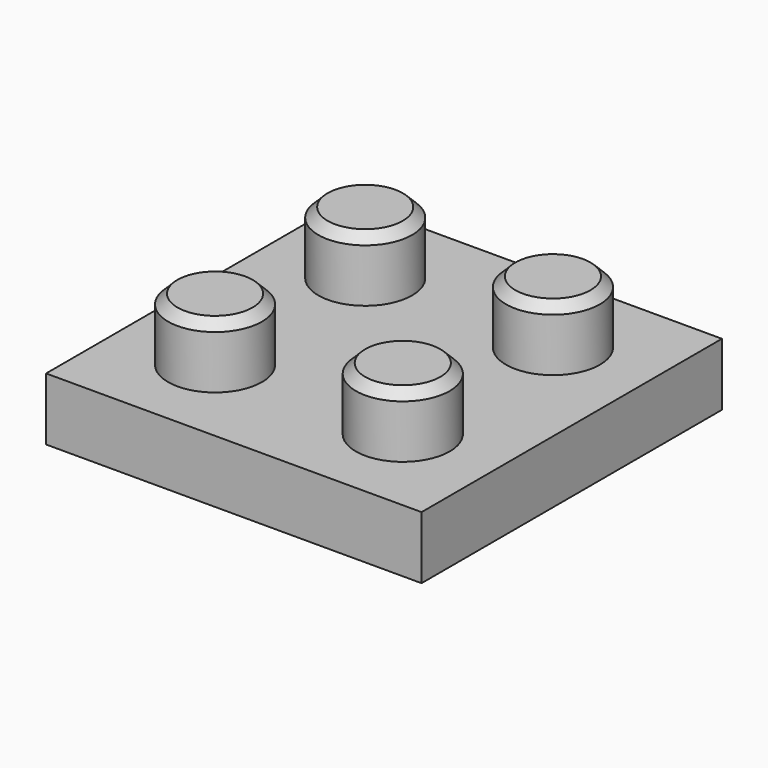
from build123d import *

# Parameters (mm, degrees)
F3_W     = 12
F3_H     = 12
F0_DEPTH = 2
F1_R     = 1.5
F4_DEPTH = 2
F5_SIZE  = 0.3
F2_T     = 1


# Not quite as in the source:
# - a shell that OpenCascade refuses in one call is made with other operations: the cavity is built on its own and cut out


with BuildPart() as f0:
    # F3 (on Top) → F0 (new body)
    with BuildSketch(Plane.XY):
        Rectangle(F3_W, F3_H)
    extrude(amount=-F0_DEPTH)

    # F1 (on Top) → F4 (join)
    with BuildSketch(Plane.XY):
        with Locations((3, 3)):
            Circle(F1_R)
        with Locations((-3, 3)):
            Circle(F1_R)
        with Locations((3, -3)):
            Circle(F1_R)
        with Locations((-3, -3)):
            Circle(F1_R)
    extrude(amount=F4_DEPTH)

    # F5
    f5_edges = [f0.edges().sort_by_distance(p)[0] for p in [
        (-4.5, 3, 2),
        (1.5, 3, 2),
        (-4.5, -3, 2),
        (1.5, -3, 2),
    ]]
    chamfer(f5_edges, length=F5_SIZE)

    # F2: shell of thickness 1, made by hand


with BuildPart() as f2_core1:
    # F2_t2: copy of F0
    add(f0.part)

    # the walls: a layer under each face that stays
    f2_faces = [f2_core1.faces().sort_by_distance(p)[0] for p in [
        (-4.5, -3, 0.85),
        (-4.35, -3, 1.85),
        (0, 0, 0),
        (-3, -3, 2),
        (0, 6, -1),
        (6, 0, -1),
        (-6, 0, -1),
        (0, -6, -1),
        (1.5, -3, 0.85),
        (-4.5, 3, 0.85),
        (1.5, 3, 0.85),
        (1.65, -3, 1.85),
        (-4.35, 3, 1.85),
        (1.65, 3, 1.85),
        (3, -3, 2),
        (-3, 3, 2),
        (3, 3, 2),
    ]]
    thicken(f2_faces, amount=-F2_T, mode=Mode.SUBTRACT)

    # F2_s3 → F2_t4 (revolve, cut)
    with BuildSketch(Plane.XZ.offset(3)):
        Polygon((-1.49, 0.01), (-2.5, 0), (-2.5, -1), (-1.5, -1), align=None)
    revolve(axis=Axis((-3, -3, 0), (0, 0, 1)), mode=Mode.SUBTRACT)

    # F2_s5 → F2_t6 (revolve, cut)
    with BuildSketch(Plane.XZ.offset(3)):
        Polygon((4.51, 0.01), (4.5, -1), (3.5, -1), (3.5, 0), align=None)
    revolve(axis=Axis((3, -3, 0), (0, 0, 1)), mode=Mode.SUBTRACT)

    # F2_s7 → F2_t8 (revolve, cut)
    with BuildSketch(Plane.XZ.offset(-3)):
        Polygon((-1.49, 0.01), (-1.5, -1), (-2.5, -1), (-2.5, 0), align=None)
    revolve(axis=Axis((-3, 3, 0), (0, 0, 1)), mode=Mode.SUBTRACT)

    # F2_s9 → F2_t10 (revolve, cut)
    with BuildSketch(Plane.XZ.offset(-3)):
        Polygon((4.51, 0.01), (4.5, -1), (3.5, -1), (3.5, 0), align=None)
    revolve(axis=Axis((3, 3, 0), (0, 0, 1)), mode=Mode.SUBTRACT)


with BuildPart() as f0_1:
    add(f0.part)

    # what is left inside the walls is the cavity
    f2_cavity = [f2_core1.part.solids().sort_by_distance(p)[0] for p in [
        (0, -1.666667, -1.99),
    ]]
    add(f2_cavity, mode=Mode.SUBTRACT)


solid = f0_1.part
